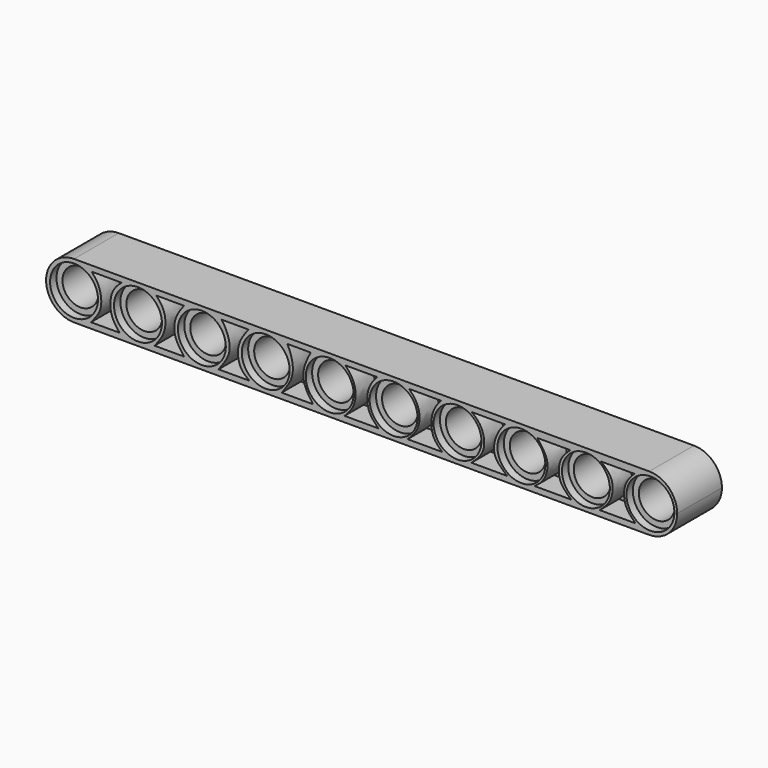
from build123d import *

# Parameters (mm, degrees)
F0_W      = 79
F0_H      = 7
F1_DEPTH  = 7
F2_R      = 3
F2_R_2    = 2.25
F2_R_3    = 2.325
F4_DEPTH  = 1
F5_DEPTH  = 8
F6_R      = 3.49999
F7_R      = 3
F7_R_2    = 2.25
F7_R_3    = 2.325
F8_DEPTH  = 1
F10_DEPTH = 3
F12_DEPTH = 3


# Not quite as in the source:
# - a fillet or chamfer is up to 0.001 mm smaller than in the source, because OpenCascade refuses the exact size


with BuildPart() as f1:
    # F0 (on Front) → F1 (new body)
    with BuildSketch(Plane.XZ):
        with Locations((-17.9342124164, 3.5)):
            Rectangle(F0_W, F0_H)
    extrude(amount=F1_DEPTH)

    # F2 (on face) → F4 (cut)
    with BuildSketch(Plane.XZ.offset(7)):
        with Locations((18.2157875836, 3.5)):
            Circle(F2_R)
        with Locations((18.2157875836, 3.5)):
            Circle(F2_R_2, mode=Mode.SUBTRACT)
        with Locations((10.1407875836, 3.5)):
            Circle(F2_R)
        with Locations((10.1407875836, 3.5)):
            Circle(F2_R_3, mode=Mode.SUBTRACT)
        with Locations((2.0657875836, 3.5)):
            Circle(F2_R)
        with Locations((2.0657875836, 3.5)):
            Circle(F2_R_2, mode=Mode.SUBTRACT)
        with Locations((-5.9342124164, 3.5)):
            Circle(F2_R)
        with Locations((-5.9342124164, 3.5)):
            Circle(F2_R_2, mode=Mode.SUBTRACT)
        with Locations((-13.9342124164, 3.5)):
            Circle(F2_R)
        with Locations((-13.9342124164, 3.5)):
            Circle(F2_R_2, mode=Mode.SUBTRACT)
        with Locations((-21.9342125942, 3.4988715429)):
            Circle(F2_R)
        with Locations((-21.9342125942, 3.4988715429)):
            Circle(F2_R_2, mode=Mode.SUBTRACT)
        with Locations((-29.9342124164, 3.5)):
            Circle(F2_R)
        with Locations((-29.9342124164, 3.5)):
            Circle(F2_R_2, mode=Mode.SUBTRACT)
        with Locations((-37.9342124164, 3.5)):
            Circle(F2_R)
        with Locations((-37.9342124164, 3.5)):
            Circle(F2_R_2, mode=Mode.SUBTRACT)
        with Locations((-45.9342124164, 3.5)):
            Circle(F2_R)
        with Locations((-45.9342124164, 3.5)):
            Circle(F2_R_2, mode=Mode.SUBTRACT)
        with Locations((-53.9342124164, 3.5)):
            Circle(F2_R)
        with Locations((-53.9342124164, 3.5)):
            Circle(F2_R_2, mode=Mode.SUBTRACT)
    extrude(amount=-F4_DEPTH, mode=Mode.SUBTRACT)

    # F2 (on face) → F5 (cut)
    with BuildSketch(Plane.XZ.offset(7)):
        with Locations((-53.9342124164, 3.5)):
            Circle(F2_R_2)
        with Locations((-45.9342124164, 3.5)):
            Circle(F2_R_2)
        with Locations((-37.9342124164, 3.5)):
            Circle(F2_R_2)
        with Locations((-29.9342124164, 3.5)):
            Circle(F2_R_2)
        with Locations((-21.9342125942, 3.4988715429)):
            Circle(F2_R_2)
        with Locations((-13.9342124164, 3.5)):
            Circle(F2_R_2)
        with Locations((-5.9342124164, 3.5)):
            Circle(F2_R_2)
        with Locations((2.0657875836, 3.5)):
            Circle(F2_R_2)
        with Locations((10.1407875836, 3.5)):
            Circle(F2_R_3)
        with Locations((18.2157875836, 3.5)):
            Circle(F2_R_2)
    extrude(amount=-F5_DEPTH, mode=Mode.SUBTRACT)

    # F6 (radius 3.5 in the source; OpenCascade refuses exactly that, so slightly less here)
    f6_edges = [f1.edges().sort_by_distance(p)[0] for p in [
        (21.565788, -3.5, 7),
        (-57.434212, -3.5, 7),
        (21.565788, -3.5, 0),
        (-57.434212, -3.5, 0),
    ]]
    fillet(f6_edges, radius=F6_R)

    # F7 (on face) → F8 (cut)
    with BuildSketch(Plane(origin=(0, 0, 0), x_dir=(-1, 0, 0), z_dir=(0, 1, 0))):
        with Locations((-18.0657875836, 3.5)):
            Circle(F7_R)
        with Locations((-18.2157875836, 3.5)):
            Circle(F7_R_2, mode=Mode.SUBTRACT)
        with Locations((-10.1407875836, 3.5)):
            Circle(F7_R)
        with Locations((-10.1407875836, 3.5)):
            Circle(F7_R_3, mode=Mode.SUBTRACT)
        with Locations((-2.0657875836, 3.5)):
            Circle(F7_R)
        with Locations((-2.0657875836, 3.5)):
            Circle(F7_R_2, mode=Mode.SUBTRACT)
        with Locations((5.9342124164, 3.5)):
            Circle(F7_R)
        with Locations((5.9342124164, 3.5)):
            Circle(F7_R_2, mode=Mode.SUBTRACT)
        with Locations((13.9342124164, 3.5)):
            Circle(F7_R)
        with Locations((13.9342124164, 3.5)):
            Circle(F7_R_2, mode=Mode.SUBTRACT)
        with Locations((21.9342125942, 3.4988715429)):
            Circle(F7_R)
        with Locations((21.9342125942, 3.4988715429)):
            Circle(F7_R_2, mode=Mode.SUBTRACT)
        with Locations((29.9342124164, 3.5)):
            Circle(F7_R)
        with Locations((29.9342124164, 3.5)):
            Circle(F7_R_2, mode=Mode.SUBTRACT)
        with Locations((37.9342124164, 3.5)):
            Circle(F7_R)
        with Locations((37.9342124164, 3.5)):
            Circle(F7_R_2, mode=Mode.SUBTRACT)
        with Locations((45.9342124164, 3.5)):
            Circle(F7_R)
        with Locations((45.9342124164, 3.5)):
            Circle(F7_R_2, mode=Mode.SUBTRACT)
        with Locations((53.9342124164, 3.5)):
            Circle(F7_R)
        with Locations((53.9342124164, 3.5)):
            Circle(F7_R_2, mode=Mode.SUBTRACT)
    extrude(amount=-F8_DEPTH, mode=Mode.SUBTRACT)

    # F9 (on face) → F10 (cut)
    with BuildSketch(Plane.XZ.offset(7)):
        with BuildLine():
            Line((-47.9664467275, 6.3172130415), (-51.7125285972, 6.3172130415))
            add(Edge.make_bspline(
                [(-51.7125285972, 6.3172130415), (-51.3649843773, 5.837141227), (-50.7675538795, 5.2700479402), (-50.2109776752, 2.5293887039), (-51.3213783514, 1.3238710323), (-51.8156946472, 0.7145957475)],
                knots=[0, 0, 0, 0, 0.2812788354, 0.6439841364, 1, 1, 1, 1], degree=3))
            Line((-51.8156946472, 0.7145957475), (-48.221193254, 0.7145957475))
            add(Edge.make_bspline(
                [(-48.221193254, 0.7145957475), (-48.6084025812, 1.1772137932), (-49.4624583626, 2.2182911477), (-49.4414214582, 4.9238155669), (-48.4364909396, 5.9389064353), (-47.9664467275, 6.3172130415)],
                knots=[0, 0, 0, 0, 0.3167233245, 0.6801474018, 1, 1, 1, 1], degree=3))
        make_face()
        with BuildLine():
            Line((-40.1561297476, 6.3172130415), (-43.6483359901, 6.3172130415))
            add(Edge.make_bspline(
                [(-43.6483359901, 6.3172130415), (-43.2945039233, 5.9536651947), (-42.4934276286, 4.9949385892), (-42.3738920069, 2.5803812392), (-43.3734632484, 1.3231382624), (-43.8596850918, 0.7145957475)],
                knots=[0, 0, 0, 0, 0.2997791553, 0.6458181247, 1, 1, 1, 1], degree=3))
            Line((-43.8596850918, 0.7145957475), (-40.1561297476, 0.7145957475))
            add(Edge.make_bspline(
                [(-40.1561297476, 6.3172130415), (-40.5813397158, 5.8259718183), (-41.3885343119, 4.6477667404), (-41.4919705398, 2.5082849281), (-40.5996000762, 1.3052095232), (-40.1561297476, 0.7145957475)],
                knots=[0, 0, 0, 0, 0.3301407402, 0.6573326151, 1, 1, 1, 1], degree=3))
        make_face()
        with BuildLine():
            Line((-32.0907179761, 6.3172130415), (-35.4607179761, 6.3172130415))
            add(Edge.make_bspline(
                [(-35.4607179761, 6.3172130415), (-35.1620063929, 5.9118194048), (-34.5863522668, 4.8749194192), (-34.2228614863, 2.870702747), (-35.2888664316, 1.4498421783), (-35.8473993838, 0.7145957475)],
                knots=[0, 0, 0, 0, 0.3001409043, 0.6211087133, 1, 1, 1, 1], degree=3))
            Line((-35.8473993838, 0.7145957475), (-31.9803993838, 0.7145957475))
            add(Edge.make_bspline(
                [(-31.9803993838, 0.7145957475), (-32.3642491763, 0.9982711551), (-33.239073779, 1.6588948311), (-33.6865963552, 4.1114030581), (-32.6483734009, 5.6273566113), (-32.0907179761, 6.3172130415)],
                knots=[0, 0, 0, 0, 0.2805819138, 0.6245252146, 1, 1, 1, 1], degree=3))
        make_face()
        with BuildLine():
            Line((-24.3019386561, 6.3172130415), (-27.2299386561, 6.3172130415))
            add(Edge.make_bspline(
                [(-27.2299386561, 6.3172130415), (-27.0069655366, 5.8971587295), (-26.570690085, 4.8219874268), (-26.4163571399, 2.7639662954), (-27.4287124335, 1.4034086137), (-27.9480591416, 0.7145957475)],
                knots=[0, 0, 0, 0, 0.2971180546, 0.6267893468, 1, 1, 1, 1], degree=3))
            Line((-27.9480591416, 0.7145957475), (-24.0260101855, 0.7145957475))
            add(Edge.make_bspline(
                [(-24.0260101855, 0.7145957475), (-24.3273745685, 1.1267151602), (-24.9727669532, 2.0204209203), (-25.4818410169, 3.941298781), (-24.7240724591, 5.5471012816), (-24.3019386561, 6.3172130415)],
                knots=[0, 0, 0, 0, 0.2969141436, 0.6192137484, 1, 1, 1, 1], degree=3))
        make_face()
        with BuildLine():
            Line((-16.0006962399, 6.3172130415), (-19.9776962399, 6.3172130415))
            add(Edge.make_bspline(
                [(-19.9776962399, 6.3172130415), (-19.528354431, 5.8645306014), (-18.645780897, 4.7277599981), (-18.6091561501, 2.2799803189), (-19.6001177261, 1.214374717), (-20.0723931193, 0.7145957475)],
                knots=[0, 0, 0, 0, 0.3256126892, 0.6695904069, 1, 1, 1, 1], degree=3))
            Line((-20.0723931193, 0.7145957475), (-15.8425774425, 0.7145957475))
            add(Edge.make_bspline(
                [(-15.8425774425, 0.7145957475), (-16.2955515719, 1.1669497281), (-17.2678436451, 2.1546382061), (-17.3111744878, 4.6651698079), (-16.4416840431, 5.8440803716), (-16.0006962399, 6.3172130415)],
                knots=[0, 0, 0, 0, 0.3212698673, 0.6708185995, 1, 1, 1, 1], degree=3))
        make_face()
        with BuildLine():
            Line((-7.9825502146, 6.3172130415), (-11.9915502146, 6.3172130415))
            add(Edge.make_bspline(
                [(-11.9915502146, 6.3172130415), (-11.5265724905, 5.8642927724), (-10.6173737621, 4.7319363409), (-10.6206415286, 2.2975703734), (-11.672581389, 1.2246670245), (-12.1809449047, 0.7145957475)],
                knots=[0, 0, 0, 0, 0.3252588499, 0.6649717928, 1, 1, 1, 1], degree=3))
            Line((-12.1809449047, 0.7145957475), (-7.8559449047, 0.7145957475))
            add(Edge.make_bspline(
                [(-7.8559449047, 0.7145957475), (-8.2976709177, 1.1256664609), (-9.2754620624, 2.0532310472), (-9.2596717803, 4.7323798429), (-8.4056080231, 5.8747658345), (-7.9825502146, 6.3172130415)],
                knots=[0, 0, 0, 0, 0.3139832374, 0.6759148374, 1, 1, 1, 1], degree=3))
        make_face()
        with BuildLine():
            add(Edge.make_bspline(
                [(-4.163, 6.3172130415), (-3.6843317219, 5.9801202472), (-2.7162025226, 5.04155925), (-2.3354969276, 2.4129201902), (-3.583554993, 1.2657348656), (-4.1947984137, 0.7145957475)],
                knots=[0, 0, 0, 0, 0.3069923844, 0.6518969691, 1, 1, 1, 1], degree=3))
            Line((-4.1947984137, 0.7145957475), (0.2872015863, 0.7145957475))
            add(Edge.make_bspline(
                [(0, 6.3172130415), (-0.3966488333, 5.8948871875), (-1.1769490989, 4.8087917918), (-1.6592654824, 2.3546992126), (-0.3573952489, 1.2510006895), (0.2872015863, 0.7145957475)],
                knots=[0, 0, 0, 0, 0.3120224204, 0.6500102037, 1, 1, 1, 1], degree=3))
            Line((0, 6.3172130415), (-4.163, 6.3172130415))
        make_face()
        with BuildLine():
            Line((8.1789931282, 6.1316555366), (4.0438743308, 6.1316555366))
            add(Edge.make_bspline(
                [(3.6966507323, 0.7145957475), (4.0938892241, 0.9922139347), (4.9710050824, 1.6103232958), (5.6984489342, 4.0314299285), (4.6094103691, 5.4139149509), (4.0438743308, 6.1316555366)],
                knots=[0, 0, 0, 0, 0.2841054952, 0.6280347397, 1, 1, 1, 1], degree=3))
            Line((3.6966507323, 0.7145957475), (8.3052571863, 0.7145957475))
            add(Edge.make_bspline(
                [(8.1789931282, 6.1316555366), (7.7275502344, 5.7199908793), (6.7709238647, 4.8474275616), (6.5915681597, 2.2180286759), (7.7390173036, 1.2098217753), (8.3052571863, 0.7145957475)],
                knots=[0, 0, 0, 0, 0.3119357713, 0.6606844568, 1, 1, 1, 1], degree=3))
        make_face()
        with BuildLine():
            Line((16.1970203562, 6.1316555366), (12.0300203562, 6.1316555366))
            add(Edge.make_bspline(
                [(11.8721909821, 0.7181218825), (12.4036125751, 1.2066834694), (13.47962177, 2.1959107921), (13.6342643795, 4.770204463), (12.5543850525, 5.68665037), (12.0300203562, 6.1316555366)],
                knots=[0, 0, 0, 0, 0.3342148924, 0.6767099832, 1, 1, 1, 1], degree=3))
            Line((11.8721909821, 0.7181218825), (16.3541909821, 0.7181218825))
            add(Edge.make_bspline(
                [(16.1970203562, 6.1316555366), (15.7571370433, 5.6570995284), (14.8436026827, 4.6715581205), (14.8610989565, 2.1575617891), (15.8657115236, 1.1890485328), (16.3541909821, 0.7181218825)],
                knots=[0, 0, 0, 0, 0.323014221, 0.6708246964, 1, 1, 1, 1], degree=3))
        make_face()
    extrude(amount=-F10_DEPTH, mode=Mode.SUBTRACT)

    # F11 (on face) → F12 (cut)
    with BuildSketch(Plane(origin=(0, 0, 0), x_dir=(-1, 0, 0), z_dir=(0, 1, 0))):
        with BuildLine():
            Line((-11.9876042008, 6.2500275671), (-16.3121186197, 6.2500275671))
            add(Edge.make_bspline(
                [(-16.3121186197, 6.2500275671), (-15.6323083821, 5.7520122992), (-14.2186466424, 4.7163922228), (-14.8985368327, 1.4881972709), (-15.9513953749, 0.9120832541), (-16.4068154991, 0.6628817646)],
                knots=[0, 0, 0, 0, 0.3445447728, 0.7164790055, 1, 1, 1, 1], degree=3))
            Line((-16.4068154991, 0.6628817646), (-11.7350779474, 0.6628817646))
            add(Edge.make_bspline(
                [(-11.7350779474, 0.6628817646), (-12.2780591157, 0.9494344135), (-13.4690780251, 1.5779822221), (-13.8268379815, 4.6210047599), (-12.5897811769, 5.7166750165), (-11.9876042008, 6.2500275671)],
                knots=[0, 0, 0, 0, 0.3007079671, 0.6595972309, 1, 1, 1, 1], degree=3))
        make_face()
        with BuildLine():
            Line((-3.8751952816, 6.2500275671), (-8.3575379103, 6.2500275671))
            add(Edge.make_bspline(
                [(-8.3575379103, 6.2500275671), (-7.7698937478, 5.8004608295), (-6.5242986215, 4.8475403839), (-6.855854158, 1.7143242318), (-7.9570245103, 0.9890477852), (-8.4522347897, 0.6628817646)],
                knots=[0, 0, 0, 0, 0.3295273496, 0.6984799419, 1, 1, 1, 1], degree=3))
            Line((-8.4522347897, 0.6628817646), (-3.4255431965, 0.6628817646))
            add(Edge.make_bspline(
                [(-3.4255431965, 0.6628817646), (-4.0629984811, 0.9600524467), (-5.4112108745, 1.5885658597), (-5.8436502159, 4.6343034287), (-4.524771226, 5.7168502437), (-3.8751952816, 6.2500275671)],
                knots=[0, 0, 0, 0, 0.3127815739, 0.6615303136, 1, 1, 1, 1], degree=3))
        make_face()
        with BuildLine():
            Line((4.0478198789, 6.2500275671), (0, 6.2500275671))
            add(Edge.make_bspline(
                [(-0.7353642723, 0.6628817646), (-0.1345785454, 0.9453734376), (1.1538342639, 1.5511899107), (1.6979325069, 4.5299096732), (0.5553312926, 5.6874402501), (0, 6.2500275671)],
                knots=[0, 0, 0, 0, 0.3099000793, 0.6645950694, 1, 1, 1, 1], degree=3))
            Line((-0.7353642723, 0.6628817646), (4.5213070698, 0.6628817646))
            add(Edge.make_bspline(
                [(4.0478198789, 6.2500275671), (3.4273435, 5.6647424313), (2.2305298878, 4.5358078878), (2.3132215694, 2.0023342002), (3.7658967288, 1.1211231782), (4.5213070698, 0.6628817646)],
                knots=[0, 0, 0, 0, 0.3406941867, 0.6571522367, 1, 1, 1, 1], degree=3))
        make_face()
        with BuildLine():
            Line((12.0970988646, 6.2500275671), (7.6147555374, 6.2500275671))
            add(Edge.make_bspline(
                [(7.1908715181, 0.6628817646), (7.8580352453, 0.90377804), (9.300882292, 1.4247543242), (9.6271874882, 4.778807646), (8.2668985023, 5.7732682308), (7.6147555374, 6.2500275671)],
                knots=[0, 0, 0, 0, 0.3092749857, 0.6688560568, 1, 1, 1, 1], degree=3))
            Line((7.1908715181, 0.6628817646), (12.6021513715, 0.6628817646))
            add(Edge.make_bspline(
                [(12.6021513715, 0.6628817646), (11.9105435431, 0.9301615118), (10.4529370881, 1.49347018), (10.140010348, 4.6449385812), (11.4530974734, 5.7218554731), (12.0970988646, 6.2500275671)],
                knots=[0, 0, 0, 0, 0.3150994532, 0.6640916688, 1, 1, 1, 1], degree=3))
        make_face()
        with BuildLine():
            Line((19.9885480106, 6.2500275671), (15.8218629658, 6.2500275671))
            add(Edge.make_bspline(
                [(15.8218629658, 6.2500275671), (16.328756772, 5.8334391098), (17.3093457885, 5.0275463157), (17.450189651, 3.3022070302), (17.1672931807, 1.5920783626), (15.8114980616, 0.9897109472), (15.0758782402, 0.6628817646)],
                knots=[0, 0, 0, 0, 0.2542595796, 0.4918666358, 0.724299808, 1, 1, 1, 1], degree=3))
            Line((15.0758782402, 0.6628817646), (20.5283872783, 0.6628817646))
            add(Edge.make_bspline(
                [(20.5283872783, 0.6628817646), (19.8476492344, 0.9339845226), (18.5212300367, 1.4622286924), (18.4260243206, 3.4848200653), (18.6900491733, 5.2190339594), (19.5608761627, 5.9104608855), (19.9885480106, 6.2500275671)],
                knots=[0, 0, 0, 0, 0.2658493826, 0.5180079591, 0.763288886, 1, 1, 1, 1], degree=3))
        make_face()
        with BuildLine():
            Line((28.0693918467, 6.2500275671), (23.6186143011, 6.2500275671))
            add(Edge.make_bspline(
                [(23.2804082334, 0.6628817646), (23.7206807712, 0.8227210271), (24.6381017723, 1.155787216), (25.4026464223, 2.7468303302), (25.4049118856, 4.1605030642), (25.001748135, 5.6642046259), (24.0802973134, 6.0544828602), (23.6186143011, 6.2500275671)],
                knots=[0, 0, 0, 0, 0.1951343553, 0.4066125871, 0.6051232256, 0.8021512441, 1, 1, 1, 1], degree=3))
            Line((23.2804082334, 0.6628817646), (28.464930132, 0.6628817646))
            add(Edge.make_bspline(
                [(28.464930132, 0.6628817646), (27.9342855798, 0.8802620905), (26.8683947446, 1.3169078568), (26.3181477848, 3.0127955829), (26.4572325401, 5.1770000845), (27.5402623369, 5.8978474175), (28.0693918467, 6.2500275671)],
                knots=[0, 0, 0, 0, 0.2394356328, 0.480947643, 0.7464096371, 1, 1, 1, 1], degree=3))
        make_face()
        with BuildLine():
            Line((36.087103188, 6.2500275671), (31.7625887692, 6.2500275671))
            add(Edge.make_bspline(
                [(31.2066450715, 0.6628817646), (31.8179663373, 0.9098029048), (33.0224772972, 1.3963215919), (33.4029142672, 3.2398958243), (33.1339699602, 5.3698631484), (32.1977836392, 5.9707157009), (31.7625887692, 6.2500275671)],
                knots=[0, 0, 0, 0, 0.25429553, 0.5010487449, 0.7680578943, 1, 1, 1, 1], degree=3))
            Line((31.2066450715, 0.6628817646), (36.5457721055, 0.6628817646))
            add(Edge.make_bspline(
                [(36.5457721055, 0.6628817646), (35.9996673064, 0.8585017932), (34.9303561063, 1.2415394224), (34.5141203705, 2.8173213693), (34.3556775477, 4.5406740781), (35.4740716738, 5.6448109564), (36.087103188, 6.2500275671)],
                knots=[0, 0, 0, 0, 0.2404348111, 0.470788092, 0.7099201706, 1, 1, 1, 1], degree=3))
        make_face()
        with BuildLine():
            Line((44.0732501447, 6.2500275671), (39.7171713412, 6.2500275671))
            add(Edge.make_bspline(
                [(39.2874889076, 0.6628817646), (39.8207992267, 0.8889442996), (40.8374665705, 1.3198948902), (41.3039190171, 2.7045651374), (41.4356489636, 4.1219405415), (40.7631520292, 5.7314748702), (40.043071267, 6.0884602577), (39.7171713412, 6.2500275671)],
                knots=[0, 0, 0, 0, 0.2137891823, 0.4075534869, 0.6086098208, 0.8228614941, 1, 1, 1, 1], degree=3))
            Line((39.2874889076, 0.6628817646), (44.5132367313, 0.6628817646))
            add(Edge.make_bspline(
                [(44.5132367313, 0.6628817646), (44.0389814524, 0.858920943), (43.1071694267, 1.2440967589), (42.5122283529, 2.5659402802), (42.4791472376, 4.5298068021), (43.1445772608, 5.7384954678), (43.7770360611, 6.0868667657), (44.0732501447, 6.2500275671)],
                knots=[0, 0, 0, 0, 0.2041965368, 0.401203312, 0.6362079576, 0.8296168439, 1, 1, 1, 1], degree=3))
        make_face()
        with BuildLine():
            Line((52.1225258708, 6.2500275671), (47.7348826826, 6.2500275671))
            add(Edge.make_bspline(
                [(47.7348826826, 6.2500275671), (48.1927169038, 5.9405407453), (49.0723878629, 5.3459006841), (49.3748396418, 3.9606785763), (49.3038219533, 2.4589938625), (48.650021307, 1.1693926818), (47.7066153205, 0.8342956898), (47.2240298986, 0.6628817646)],
                knots=[0, 0, 0, 0, 0.2087211685, 0.4010315131, 0.6051097626, 0.7979997217, 1, 1, 1, 1], degree=3))
            Line((47.2240298986, 0.6628817646), (52.6971556246, 0.6628817646))
            add(Edge.make_bspline(
                [(52.6971556246, 0.6628817646), (52.1467775073, 0.7893246685), (51.0998852757, 1.0298358546), (50.5885413455, 2.2996418839), (50.2406461496, 4.0421064459), (50.8925605063, 5.3089377877), (51.7029895985, 5.9290256029), (52.1225258708, 6.2500275671)],
                knots=[0, 0, 0, 0, 0.2048200025, 0.3895948307, 0.6058204744, 0.7959443826, 1, 1, 1, 1], degree=3))
        make_face()
    extrude(amount=-F12_DEPTH, mode=Mode.SUBTRACT)


solid = f1.part
